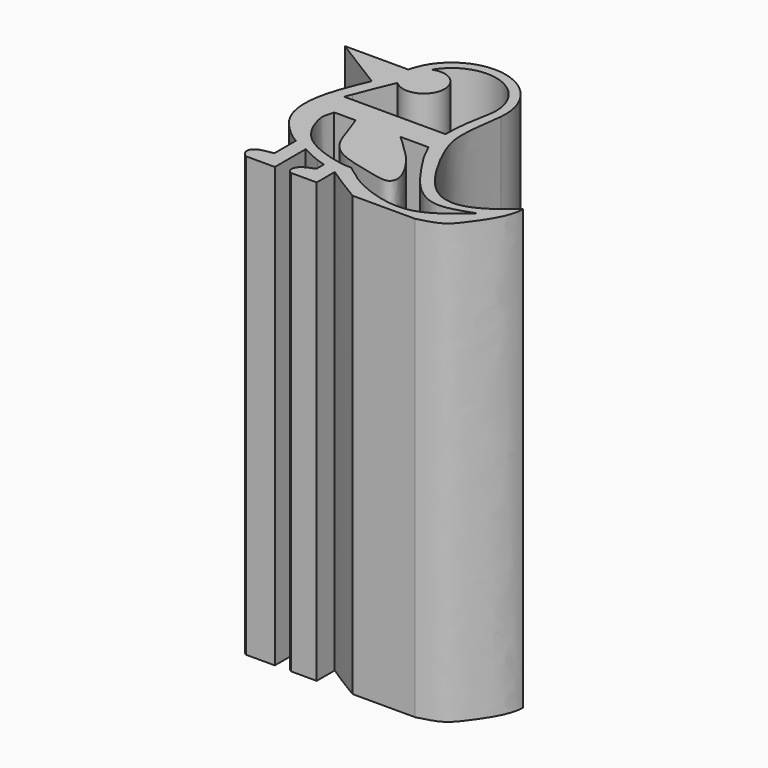
from build123d import *

# Parameters (mm, degrees)
F1_DEPTH = 25.4


with BuildPart() as f1:
    # F0 (on Top) → F1 (new body)
    with BuildSketch(Plane.XY):
        with BuildLine():
            add(Edge.make_bspline(
                [(-20.3382612037, 35.8313347316), (-20.4450111683, 34.9358050979), (-20.6956038594, 33.4295119082), (-20.4520091655, 31.8862395133), (-19.0946101464, 29.3170291608), (-17.8111689332, 27.9825807986), (-16.4324991862, 27.7419027231), (-15.0794261509, 28.4031430479), (-14.2998902994, 29.0480302806), (-13.904822059, 29.3747521937)],
                knots=[0, 0, 0, 0, 0.1653037084, 0.2975853738, 0.4776663545, 0.6214793879, 0.7401281155, 0.8679936909, 1, 1, 1, 1], degree=3))
            ThreePointArc((-20.3382612037, 35.8313347316), (-22.9562506508, 39.2154729726), (-26.4925179517, 36.8069310992))
            Line((-26.4925179517, 36.8069310992), (-26.5022447151, 36.8069310992))
            add(Edge.make_bspline(
                [(-26.5022447151, 36.8069310992), (-26.5819130783, 36.1808218197), (-26.8148696335, 35.5395069688), (-27.0769987784, 34.8878260057)],
                knots=[0, 0, 0, 0, 0.1885118186, 0.1885118186, 0.1885118186, 0.1885118186], degree=3))
            add(Edge.make_bspline(
                [(-27.0769987784, 34.8878260057), (-27.3225638709, 34.2773250402), (-28.1095019562, 32.4792264142), (-28.326739249, 29.6855427651), (-26.1714588887, 28.1815095827), (-26.1127384914, 28.2024321762), (-26.1040050536, 28.2070487738)],
                knots=[0.1885118186, 0.1885118186, 0.1885118186, 0.1885118186, 0.365111495, 0.7010109468, 0.966132419, 1, 1, 1, 1], degree=3))
            Line((-26.1040050536, 28.2070487738), (-26.1040050536, 26.6290362924))
            add(Edge.make_bspline(
                [(-26.1040050536, 26.6290362924), (-26.50786087, 26.5663915047), (-27.1725068155, 26.4619725648), (-27.2738381155, 25.8754369894), (-27.0432563694, 25.6828019605), (-26.9273165613, 25.5914572626)],
                knots=[0, 0, 0, 0, 0.4399850766, 0.7208050242, 1, 1, 1, 1], degree=3))
            Line((-26.9273165613, 25.5914572626), (-25.2463910729, 25.5914572626))
            Line((-25.2463910729, 25.5914572626), (-25.2463910729, 25.771420449))
            add(Edge.make_bspline(
                [(-25.2463910729, 26.6290362924), (-25.2463910729, 26.3431643446), (-25.2463910729, 26.0572923968), (-25.2463910729, 25.771420449)],
                knots=[0, 0, 0, 0, 0.8576158434, 0.8576158434, 0.8576158434, 0.8576158434], degree=3))
            Line((-25.2463910729, 26.6290362924), (-25.2463910729, 27.8230719268))
            add(Edge.make_bspline(
                [(-25.2463910729, 27.8230719268), (-25.0259420337, 27.7154537877), (-24.6676994209, 27.5206856825), (-24.3170251754, 27.3869259749), (-24.1801459342, 27.3284353316)],
                knots=[0, 0, 0, 0, 0.5361258831, 1, 1, 1, 1], degree=3))
            add(Edge.make_bspline(
                [(-24.1801459342, 27.3284353316), (-24.0093345443, 27.27341714), (-23.8385231545, 27.2183989485), (-23.6677117646, 27.163380757)],
                knots=[0, 0, 0, 0, 0.5383602798, 0.5383602798, 0.5383602798, 0.5383602798], degree=3))
            Line((-23.6677117646, 27.163380757), (-23.6677117646, 26.6290362924))
            add(Edge.make_bspline(
                [(-23.6677117646, 26.6290362924), (-23.8486112672, 26.5599101731), (-24.1839606126, 26.4320640725), (-24.5156260038, 26.159992966), (-24.5633962408, 25.7689710346), (-24.4001932512, 25.6449799988), (-24.3170251754, 25.5914572626)],
                knots=[0, 0, 0, 0, 0.3002488033, 0.5568370832, 0.7879058054, 1, 1, 1, 1], degree=3))
            Line((-24.3170251754, 25.5914572626), (-22.8249467909, 25.5914572626))
            Line((-22.8249467909, 25.5914572626), (-22.8249467909, 26.6290362924))
            Line((-22.8249467909, 26.6290362924), (-22.8249467909, 26.8962085247))
            add(Edge.make_bspline(
                [(-22.8249467909, 26.8962085247), (-22.5713066122, 26.7276144339), (-22.0028986749, 26.3497948791), (-21.195758956, 25.8617321727), (-20.7487884909, 25.5914572626)],
                knots=[0, 0, 0, 0, 0.446229129, 1, 1, 1, 1], degree=3))
            add(Edge.make_bspline(
                [(-20.7487884909, 25.5914572626), (-20.6447985865, 25.5914572626), (-20.2492258993, 25.5914572626), (-18.450568256, 25.5914572626), (-17.1247497201, 25.5914572626)],
                knots=[0, 0, 0, 0, 0.26288444, 1, 1, 1, 1], degree=3))
            add(Edge.make_bspline(
                [(-17.1247497201, 25.5914572626), (-16.7304722372, 25.6996906729), (-15.7777839891, 25.9141544333), (-14.9929303539, 26.9268449842), (-13.8994103483, 28.4848795653), (-13.904822059, 29.3747521937)],
                knots=[0, 0, 0, 0, 0.2906764391, 0.5819576128, 1, 1, 1, 1], degree=3))
        make_face()
        with BuildLine():
            Line((-22.6698517799, 31.4386411512), (-21.0337025163, 31.4386411512))
            add(Edge.make_bspline(
                [(-21.0337025163, 31.4386411512), (-20.8902139077, 31.1323245172), (-20.5931961172, 30.4982568329), (-19.948402137, 29.5555814465), (-18.8033343493, 27.8881326011), (-17.2274089816, 27.0450525014), (-15.957345343, 27.5098448702), (-15.2919646353, 27.753347531)],
                knots=[0, 0, 0, 0, 0.1624195956, 0.3362044547, 0.5652089994, 0.772214923, 1, 1, 1, 1], degree=3))
            add(Edge.make_bspline(
                [(-21.6075759381, 27.0229037851), (-21.2921258199, 26.8415588149), (-20.5169526668, 26.3959297147), (-17.7138645688, 25.6180239971), (-16.1224872042, 27.0210982904), (-15.2919646353, 27.753347531)],
                knots=[0, 0, 0, 0, 0.2470261496, 0.6070311225, 1, 1, 1, 1], degree=3))
            add(Edge.make_bspline(
                [(-22.4931623569, 27.695426443), (-22.1939764772, 27.4138094891), (-21.9067618178, 27.3045207391), (-21.6075759381, 27.0229037851)],
                knots=[0, 0, 0, 0, 1.1120027116, 1.1120027116, 1.1120027116, 1.1120027116], degree=3))
            add(Edge.make_bspline(
                [(-26.4862797308, 31.4386411512), (-26.6259402071, 30.9096946323), (-26.6783712453, 30.7603514323), (-26.3997968938, 29.6282073765), (-25.4490435424, 28.3489615598), (-23.4013330994, 27.741539672), (-22.7768510314, 27.6881511475), (-22.4931623569, 27.695426443)],
                knots=[0, 0, 0, 0, 0.1625930825, 0.3386475555, 0.5683904873, 0.8284157553, 1, 1, 1, 1], degree=3))
            Line((-26.4862797308, 31.4386411512), (-25.2517569845, 31.4386411512))
            add(Edge.make_bspline(
                [(-25.2517569845, 31.4386411512), (-25.081467778, 31.0305250114), (-24.8474412541, 30.2487875622), (-24.1954181543, 28.3934750124), (-21.7113422378, 27.9363030082), (-20.387241461, 27.5366712966), (-20.0063896806, 28.2928764563), (-21.0142921465, 29.9153907257), (-21.7761724236, 30.57659681), (-22.3482616293, 31.1915019356), (-22.6698517799, 31.4386411512)],
                knots=[0, 0, 0, 0, 0.1205697372, 0.2621090922, 0.4299069649, 0.5482397404, 0.6270841, 0.770560927, 0.8827722027, 1, 1, 1, 1], degree=3))
        make_face(mode=Mode.SUBTRACT)
        with BuildLine():
            ThreePointArc((-25.654328987, 37.4647304416), (-22.4769363023, 38.524071468), (-20.9311007312, 35.5528057326))
            add(Edge.make_bspline(
                [(-20.9311007312, 35.5528057326), (-21.0622856997, 34.8308373887), (-21.2217965052, 33.9606944337), (-21.2295446647, 33.070501474), (-21.2261399372, 32.9183340073)],
                knots=[0, 0, 0, 0, 0.3234940663, 0.3900255115, 0.3900255115, 0.3900255115, 0.3900255115], degree=3))
            Line((-21.2261399372, 32.9183340073), (-22.6698517799, 32.9183340073))
            Line((-22.6698517799, 32.9183340073), (-25.2517569845, 32.9183340073))
            Line((-25.2517569845, 32.9183340073), (-26.4331996441, 32.9183340073))
            Line((-26.4331996441, 32.9183340073), (-27.1009020507, 32.9183340073))
            Line((-27.1009020507, 32.9183340073), (-26.9288700074, 33.3305411041))
            add(Edge.make_bspline(
                [(-26.056057546, 35.4814045858), (-26.2491927806, 35.0294793202), (-26.5989642929, 34.2109348307), (-26.8267870878, 33.6029618535), (-26.9288700074, 33.3305411041)],
                knots=[0.0013306924, 0.0013306924, 0.0013306924, 0.0013306924, 0.5525158988, 1, 1, 1, 1], degree=3))
            ThreePointArc((-26.056057546, 35.4814045858), (-24.0453939283, 36.1064872676), (-25.654328987, 37.4647304416))
        make_face(mode=Mode.SUBTRACT)
        with BuildLine():
            add(Edge.make_bspline(
                [(-26.5022447151, 36.8069310992), (-26.5819130783, 36.1808218197), (-26.8148696335, 35.5395069688), (-27.0769987784, 34.8878260057)],
                knots=[0, 0, 0, 0, 0.1885118186, 0.1885118186, 0.1885118186, 0.1885118186], degree=3))
            Line((-26.5022447151, 36.8069310992), (-30.1676038653, 36.8069310992))
            Line((-30.1676038653, 36.8069310992), (-27.0769987784, 34.8878260057))
        make_face()
    extrude(amount=F1_DEPTH)


solid = f1.part
